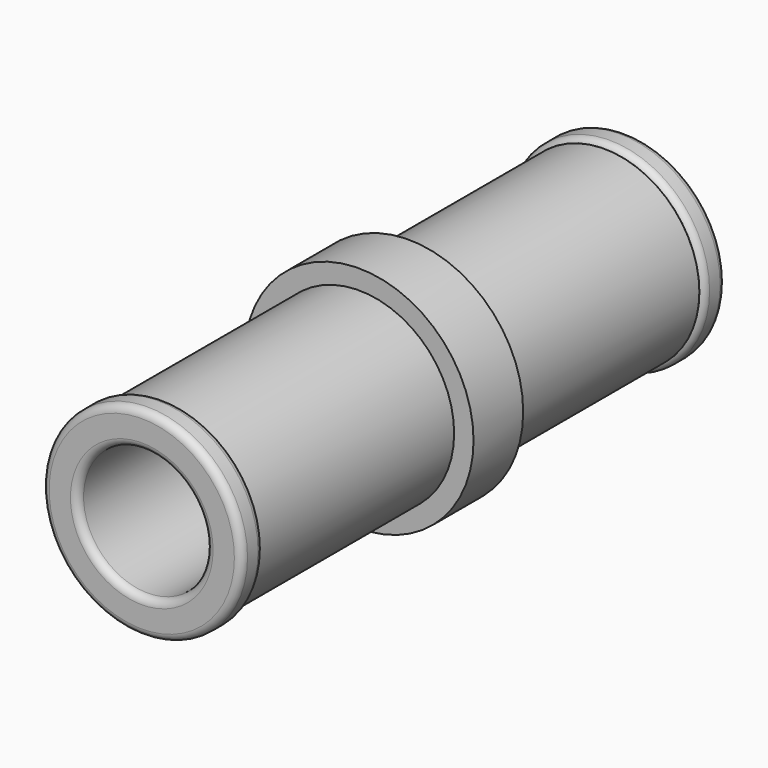
from build123d import *

# Parameters (mm, degrees)
F0_R     = 2.95
F0_R_2   = 2.575
F1_DEPTH = 0.8
F0_R_3   = 2.45
F2_DEPTH = 0.8
F0_R_4   = 1.65
F3_DEPTH = 7.8
F4_DEPTH = 7.8
F5_DEPTH = 7.1
F6_DEPTH = 7.8
F7_DEPTH = 0.8


# Not quite as in the source:
# - a fillet or chamfer that OpenCascade refuses, or shapes differently, is made with other operations: its cross-section is extruded or revolved along the edge and cut away or added


with BuildPart() as f1:
    # F0 (on Front) → F1 (new body)
    with BuildSketch(Plane.XZ):
        with Locations((-40.3700359166, 25.8709397167)):
            Circle(F0_R)
        with Locations((-40.3700359166, 25.8709397167)):
            Circle(F0_R_2, mode=Mode.SUBTRACT)
    extrude(amount=F1_DEPTH)

    # F0 (on Front) → F2 (join)
    with BuildSketch(Plane.XZ):
        with Locations((-40.3700359166, 25.8709397167)):
            Circle(F0_R_2)
        with Locations((-40.3700359166, 25.8709397167)):
            Circle(F0_R_3, mode=Mode.SUBTRACT)
    extrude(amount=F2_DEPTH)

    # F0 (on Front) → F3 (join)
    with BuildSketch(Plane.XZ):
        with Locations((-40.3700359166, 25.8709397167)):
            Circle(F0_R_3)
        with Locations((-40.3700359166, 25.8709397167)):
            Circle(F0_R_4, mode=Mode.SUBTRACT)
    extrude(amount=F3_DEPTH)

    # F0 (on Front) → F4 (join)
    with BuildSketch(Plane.XZ):
        with Locations((-40.3700359166, 25.8709397167)):
            Circle(F0_R_2)
        with Locations((-40.3700359166, 25.8709397167)):
            Circle(F0_R_3, mode=Mode.SUBTRACT)
    extrude(amount=F4_DEPTH)

    # F0 (on Front) → F5 (cut)
    with BuildSketch(Plane.XZ):
        with Locations((-40.3700359166, 25.8709397167)):
            Circle(F0_R_2)
        with Locations((-40.3700359166, 25.8709397167)):
            Circle(F0_R_3, mode=Mode.SUBTRACT)
    extrude(amount=F5_DEPTH, mode=Mode.SUBTRACT)

    # F0 (on Front) → F6 (join)
    with BuildSketch(Plane.XZ):
        with Locations((-40.3700359166, 25.8709397167)):
            Circle(F0_R_3)
        with Locations((-40.3700359166, 25.8709397167)):
            Circle(F0_R_4, mode=Mode.SUBTRACT)
    extrude(amount=-F6_DEPTH)

    # F0 (on Front) → F7 (join)
    with BuildSketch(Plane.XZ):
        with Locations((-40.3700359166, 25.8709397167)):
            Circle(F0_R)
        with Locations((-40.3700359166, 25.8709397167)):
            Circle(F0_R_2, mode=Mode.SUBTRACT)
        with Locations((-40.3700359166, 25.8709397167)):
            Circle(F0_R_2)
        with Locations((-40.3700359166, 25.8709397167)):
            Circle(F0_R_3, mode=Mode.SUBTRACT)
    extrude(amount=-F7_DEPTH)

    # F8: F1 across plane


with BuildPart() as f1_1:
    add(f1.part)
    add(f1.part.mirror(Plane.XZ))

    # F9: fillet of radius 0.2 on 6 edges, made by hand

    # F9_s1 → F9_t2 (revolve, cut)
    with BuildSketch(Plane.XY.offset(25.8709397167)):
        with BuildLine():
            ThreePointArc((-38.5190702311, -7.8004), (-38.6614572728, -7.7414213562), (-38.7204359166, -7.5990343146))
            Line((-38.7204359166, -7.5990343146), (-38.7405724851, -7.5990343146))
            ThreePointArc((-38.7405724851, -7.5990343146), (-38.7401724851, -7.6995171573), (-38.7401724851, -7.8))
            Line((-38.7401724851, -7.8), (-38.7200359166, -7.8201365685))
            ThreePointArc((-38.7200359166, -7.8201365685), (-38.6195530739, -7.8201365685), (-38.5190702311, -7.8205365685))
            Line((-38.5190702311, -7.8205365685), (-38.5190702311, -7.8004))
        make_face()
    revolve(axis=Axis((-40.3700359166, -7.8, 25.8709397167), (0, -1, 0)), mode=Mode.SUBTRACT)

    # F9_s3 → F9_t4 (revolve, cut)
    with BuildSketch(Plane.XY.offset(25.8709397167)):
        with BuildLine():
            ThreePointArc((-37.7946359166, -7.5990343146), (-37.8536145603, -7.7414213562), (-37.996001602, -7.8004))
            Line((-37.996001602, -7.8004), (-37.996001602, -7.8205365685))
            ThreePointArc((-37.996001602, -7.8205365685), (-37.8955187593, -7.8201365685), (-37.7950359166, -7.8201365685))
            Line((-37.7950359166, -7.8201365685), (-37.774899348, -7.8))
            ThreePointArc((-37.774899348, -7.8), (-37.774899348, -7.6995171573), (-37.774499348, -7.5990343146))
            Line((-37.774499348, -7.5990343146), (-37.7946359166, -7.5990343146))
        make_face()
    revolve(axis=Axis((-40.3700359166, -7.8, 25.8709397167), (0, -1, 0)), mode=Mode.SUBTRACT)

    # F9_s5 → F9_t6 (revolve, cut)
    with BuildSketch(Plane.XY.offset(25.8709397167)):
        with BuildLine():
            ThreePointArc((-37.9198847153, -7.0996296783), (-37.828855755, -7.173758828), (-37.7946359166, -7.286054888))
            Line((-37.7946359166, -7.286054888), (-37.774499348, -7.286054888))
            ThreePointArc((-37.774499348, -7.286054888), (-37.774899348, -7.193027444), (-37.774899348, -7.1))
            Line((-37.774899348, -7.1), (-37.7950359166, -7.0798634315))
            ThreePointArc((-37.7950359166, -7.0798634315), (-37.8574603159, -7.0798634315), (-37.9122730266, -7.0809871573))
            Line((-37.9122730266, -7.0809871573), (-37.9198847153, -7.0996296783))
        make_face()
    revolve(axis=Axis((-40.3700359166, -7.1, 25.8709397167), (0, -1, 0)), mode=Mode.SUBTRACT)

    # F9_s7 → F9_t8 (revolve, cut)
    with BuildSketch(Plane.XY.offset(25.8709397167)):
        with BuildLine():
            ThreePointArc((-37.996001602, 7.8004), (-37.8536145603, 7.7414213562), (-37.7946359166, 7.5990343146))
            Line((-37.7946359166, 7.5990343146), (-37.774499348, 7.5990343146))
            ThreePointArc((-37.774499348, 7.5990343146), (-37.774899348, 7.6995171573), (-37.774899348, 7.8))
            Line((-37.774899348, 7.8), (-37.7950359166, 7.8201365685))
            ThreePointArc((-37.7950359166, 7.8201365685), (-37.8955187593, 7.8201365685), (-37.996001602, 7.8205365685))
            Line((-37.996001602, 7.8205365685), (-37.996001602, 7.8004))
        make_face()
    revolve(axis=Axis((-40.3700359166, 7.8, 25.8709397167), (0, -1, 0)), mode=Mode.SUBTRACT)

    # F9_s9 → F9_t10 (revolve, cut)
    with BuildSketch(Plane.XY.offset(25.8709397167)):
        with BuildLine():
            ThreePointArc((-37.9198847153, 7.0996296783), (-37.828855755, 7.173758828), (-37.7946359166, 7.286054888))
            Line((-37.7946359166, 7.286054888), (-37.774499348, 7.286054888))
            ThreePointArc((-37.774499348, 7.286054888), (-37.774899348, 7.193027444), (-37.774899348, 7.1))
            Line((-37.774899348, 7.1), (-37.7950359166, 7.0798634315))
            ThreePointArc((-37.7950359166, 7.0798634315), (-37.8574603159, 7.0798634315), (-37.9122730266, 7.0809871573))
            Line((-37.9122730266, 7.0809871573), (-37.9198847153, 7.0996296783))
        make_face()
    revolve(axis=Axis((-40.3700359166, 7.1, 25.8709397167), (0, -1, 0)), mode=Mode.SUBTRACT)

    # F9_s11 → F9_t12 (revolve, cut)
    with BuildSketch(Plane.XY.offset(25.8709397167)):
        with BuildLine():
            ThreePointArc((-38.7204359166, 7.5990343146), (-38.6614572728, 7.7414213562), (-38.5190702311, 7.8004))
            Line((-38.5190702311, 7.8004), (-38.5190702311, 7.8205365685))
            ThreePointArc((-38.5190702311, 7.8205365685), (-38.6195530739, 7.8201365685), (-38.7200359166, 7.8201365685))
            Line((-38.7200359166, 7.8201365685), (-38.7401724851, 7.8))
            ThreePointArc((-38.7401724851, 7.8), (-38.7401724851, 7.6995171573), (-38.7405724851, 7.5990343146))
            Line((-38.7405724851, 7.5990343146), (-38.7204359166, 7.5990343146))
        make_face()
    revolve(axis=Axis((-40.3700359166, 7.8, 25.8709397167), (0, -1, 0)), mode=Mode.SUBTRACT)


solid = f1_1.part
